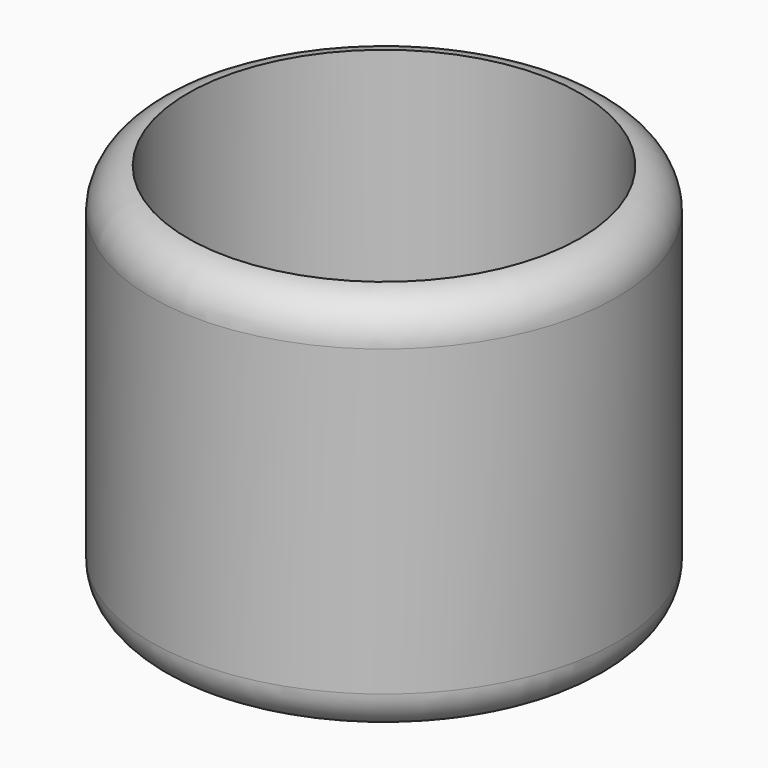
from build123d import *

# Parameters (mm, degrees)
F0_R     = 11.5
F1_DEPTH = 19
F2_T     = -1.8


# Not quite as in the source:
# - a fillet or chamfer that OpenCascade refuses, or shapes differently, is made with other operations: its cross-section is extruded or revolved along the edge and cut away or added


with BuildPart() as f1:
    # F0 (on Top) → F1 (new body)
    with BuildSketch(Plane.XY):
        Circle(F0_R)
    extrude(amount=-F1_DEPTH)

    # F2
    f2_openings = [f1.faces().sort_by_distance(p)[0] for p in [
        (0, 0, 0),
    ]]
    offset(amount=F2_T, openings=f2_openings)

    # F3: fillet of radius 2 on 2 edges, made by hand

    # F3_s1 → F3_t2 (revolve, cut)
    with BuildSketch(Plane.XZ):
        with BuildLine():
            ThreePointArc((11.5, -17), (10.9142135624, -18.4142135624), (9.5, -19))
            Line((9.5, -19), (11.5, -19))
            Line((11.5, -19), (11.5, -17))
        make_face()
    revolve(axis=Axis((0, 0, -19), (0, 0, 1)), mode=Mode.SUBTRACT)

    # F3_s3 → F3_t4 (revolve, cut)
    with BuildSketch(Plane.XZ):
        with BuildLine():
            ThreePointArc((11.5, -1.9899748742), (10.9832396974, -0.6483340877), (9.7, 0))
            Line((9.7, 0), (11.5, 0))
            Line((11.5, 0), (11.5, -1.9899748742))
        make_face()
    revolve(axis=Axis((0, 0, 0), (0, 0, 1)), mode=Mode.SUBTRACT)


solid = f1.part
